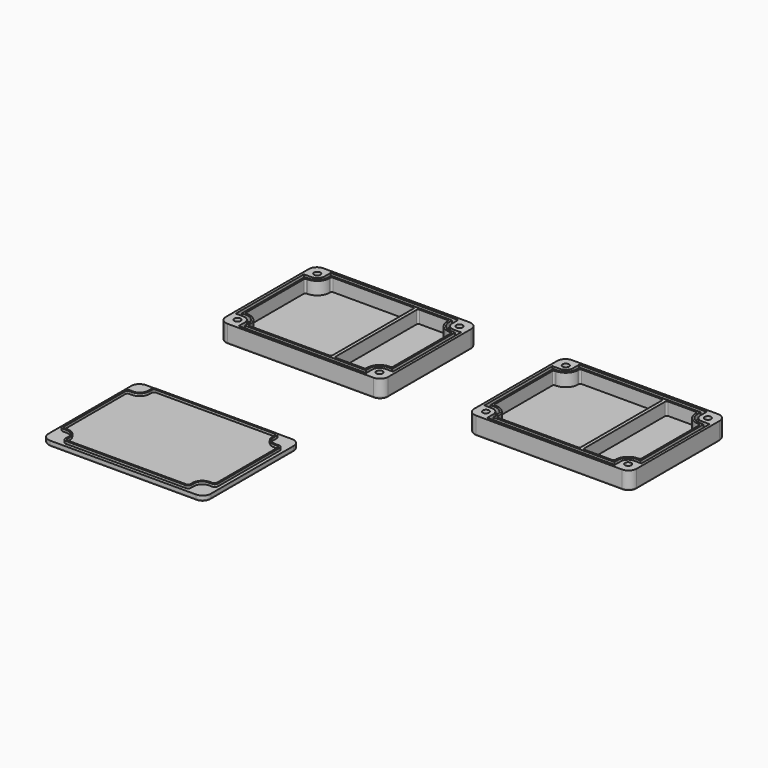
from build123d import *

# Parameters (mm, degrees)
F0_R      = 1.95
F1_DEPTH  = 11
F2_DEPTH  = 8
F3_DEPTH  = 3.2
F4_R      = 1.25
F5_DEPTH  = 3.2
F4_W      = 2
F4_H      = 66.4
F6_DEPTH  = 4.7
F4_R_2    = 2.75
F7_DEPTH  = 3.2
F8_DEPTH  = 3.2
F9_DEPTH  = 3.2
F10_R     = 1
F10_2_R   = 1
F12_R     = 3.65
F12_R_2   = 1.95
F13_DEPTH = 3.7
F17_DEPTH = 1.5
F18_DEPTH = 1.5
F19_R     = 2


# Not quite as in the source:
# - two fillets or chamfers of one size are made in one step


with BuildPart() as f1:
    # F0 (on Top) → F1 (new body)
    with BuildSketch(Plane.XY):
        with BuildLine():
            Line((56.8, 36.8), (-32.8, 36.8))
            ThreePointArc((-32.8, 36.8), (-36.3355339059, 35.3355339059), (-37.8, 31.8))
            Line((-37.8, 31.8), (-37.8, -31.8))
            ThreePointArc((-37.8, -31.8), (-36.3355339059, -35.3355339059), (-32.8, -36.8))
            Line((-32.8, -36.8), (56.8, -36.8))
            ThreePointArc((56.8, -36.8), (60.3355339059, -35.3355339059), (61.8, -31.8))
            Line((61.8, -31.8), (61.8, 31.8))
            ThreePointArc((61.8, 31.8), (60.3355339059, 35.3355339059), (56.8, 36.8))
        make_face()
        with Locations((-31.6, -30.6)):
            Circle(F0_R, mode=Mode.SUBTRACT)
        with Locations((55.6, -30.6)):
            Circle(F0_R, mode=Mode.SUBTRACT)
        with BuildLine():
            Line((51.1, -35.2), (-27.1, -35.2))
            Line((-27.1, -35.2), (-27.1, -30.6))
            ThreePointArc((-27.1, -30.6), (-28.4180194847, -27.4180194847), (-31.6, -26.1))
            Line((-31.6, -26.1), (-36.2, -26.1))
            Line((-36.2, -26.1), (-36.2, 26.1))
            Line((-36.2, 26.1), (-31.6, 26.1))
            ThreePointArc((-31.6, 26.1), (-28.4180194847, 27.4180194847), (-27.1, 30.6))
            Line((-27.1, 30.6), (-27.1, 35.2))
            Line((-27.1, 35.2), (51.1, 35.2))
            Line((51.1, 35.2), (51.1, 30.6))
            ThreePointArc((51.1, 30.6), (52.4180194847, 27.4180194847), (55.6, 26.1))
            Line((55.6, 26.1), (60.2, 26.1))
            Line((60.2, 26.1), (60.2, -26.1))
            Line((60.2, -26.1), (55.6, -26.1))
            ThreePointArc((55.6, -26.1), (52.4180194847, -27.4180194847), (51.1, -30.6))
            Line((51.1, -30.6), (51.1, -35.2))
        make_face(mode=Mode.SUBTRACT)
        with Locations((-31.6, 30.6)):
            Circle(F0_R, mode=Mode.SUBTRACT)
        with Locations((55.6, 30.6)):
            Circle(F0_R, mode=Mode.SUBTRACT)
    extrude(amount=F1_DEPTH)



with BuildPart() as f1b:
    # F0 (on Top) → F1, piece 2 (new body)
    with BuildSketch(Plane.XY):
        with BuildLine():
            Line((49.1, 33.1), (-25.1, 33.1))
            Line((-25.1, 33.1), (-25.1, 30.6))
            ThreePointArc((-25.1, 30.6), (-27.0038059223, 26.0038059223), (-31.6, 24.1))
            Line((-31.6, 24.1), (-34.1, 24.1))
            Line((-34.1, 24.1), (-34.1, -24.1))
            Line((-34.1, -24.1), (-31.6, -24.1))
            ThreePointArc((-31.6, -24.1), (-27.0038059223, -26.0038059223), (-25.1, -30.6))
            Line((-25.1, -30.6), (-25.1, -33.1))
            Line((-25.1, -33.1), (49.1, -33.1))
            Line((49.1, -33.1), (49.1, -30.6))
            ThreePointArc((49.1, -30.6), (51.0038059223, -26.0038059223), (55.6, -24.1))
            Line((55.6, -24.1), (58.1, -24.1))
            Line((58.1, -24.1), (58.1, 24.1))
            Line((58.1, 24.1), (55.6, 24.1))
            ThreePointArc((55.6, 24.1), (51.0038059223, 26.0038059223), (49.1, 30.6))
            Line((49.1, 30.6), (49.1, 33.1))
        make_face()
        with BuildLine():
            Line((-24, 30.6), (-24, 32))
            Line((-24, 32), (27, 32))
            Line((27, 32), (27, -32))
            Line((27, -32), (-24, -32))
            Line((-24, -32), (-24, -30.6))
            ThreePointArc((-24, -30.6), (-26.225988463, -25.225988463), (-31.6, -23))
            Line((-31.6, -23), (-33, -23))
            Line((-33, -23), (-33, 23))
            Line((-33, 23), (-31.6, 23))
            ThreePointArc((-31.6, 23), (-26.225988463, 25.225988463), (-24, 30.6))
        make_face(mode=Mode.SUBTRACT)
        with BuildLine():
            Line((55.6, 23), (57, 23))
            Line((57, 23), (57, -23))
            Line((57, -23), (55.6, -23))
            ThreePointArc((55.6, -23), (50.225988463, -25.225988463), (48, -30.6))
            Line((48, -30.6), (48, -32))
            Line((48, -32), (29, -32))
            Line((29, -32), (29, 32))
            Line((29, 32), (48, 32))
            Line((48, 32), (48, 30.6))
            ThreePointArc((48, 30.6), (50.225988463, 25.225988463), (55.6, 23))
        make_face(mode=Mode.SUBTRACT)
    extrude(amount=F1_DEPTH)


with BuildPart() as f1_1:
    add(f1.part)

    add(f1b.part)  # F2 merges F1b
    # F0 (on Top) → F2 (join)
    with BuildSketch(Plane.XY):
        with BuildLine():
            Line((-27.1, -30.6), (-27.1, -35.2))
            Line((-27.1, -35.2), (51.1, -35.2))
            Line((51.1, -35.2), (51.1, -30.6))
            ThreePointArc((51.1, -30.6), (52.4180194847, -27.4180194847), (55.6, -26.1))
            Line((55.6, -26.1), (60.2, -26.1))
            Line((60.2, -26.1), (60.2, 26.1))
            Line((60.2, 26.1), (55.6, 26.1))
            ThreePointArc((55.6, 26.1), (52.4180194847, 27.4180194847), (51.1, 30.6))
            Line((51.1, 30.6), (51.1, 35.2))
            Line((51.1, 35.2), (-27.1, 35.2))
            Line((-27.1, 35.2), (-27.1, 30.6))
            ThreePointArc((-27.1, 30.6), (-28.4180194847, 27.4180194847), (-31.6, 26.1))
            Line((-31.6, 26.1), (-36.2, 26.1))
            Line((-36.2, 26.1), (-36.2, -26.1))
            Line((-36.2, -26.1), (-31.6, -26.1))
            ThreePointArc((-31.6, -26.1), (-28.4180194847, -27.4180194847), (-27.1, -30.6))
        make_face()
        with BuildLine():
            Line((-25.1, 30.6), (-25.1, 33.1))
            Line((-25.1, 33.1), (49.1, 33.1))
            Line((49.1, 33.1), (49.1, 30.6))
            ThreePointArc((49.1, 30.6), (51.0038059223, 26.0038059223), (55.6, 24.1))
            Line((55.6, 24.1), (58.1, 24.1))
            Line((58.1, 24.1), (58.1, -24.1))
            Line((58.1, -24.1), (55.6, -24.1))
            ThreePointArc((55.6, -24.1), (51.0038059223, -26.0038059223), (49.1, -30.6))
            Line((49.1, -30.6), (49.1, -33.1))
            Line((49.1, -33.1), (-25.1, -33.1))
            Line((-25.1, -33.1), (-25.1, -30.6))
            ThreePointArc((-25.1, -30.6), (-27.0038059223, -26.0038059223), (-31.6, -24.1))
            Line((-31.6, -24.1), (-34.1, -24.1))
            Line((-34.1, -24.1), (-34.1, 24.1))
            Line((-34.1, 24.1), (-31.6, 24.1))
            ThreePointArc((-31.6, 24.1), (-27.0038059223, 26.0038059223), (-25.1, 30.6))
        make_face(mode=Mode.SUBTRACT)
    extrude(amount=F2_DEPTH)

    # F0 (on Top) → F3 (join)
    with BuildSketch(Plane.XY):
        with BuildLine():
            Line((57, -23), (57, 23))
            Line((57, 23), (55.6, 23))
            ThreePointArc((55.6, 23), (50.225988463, 25.225988463), (48, 30.6))
            Line((48, 30.6), (48, 32))
            Line((48, 32), (29, 32))
            Line((29, 32), (29, -32))
            Line((29, -32), (48, -32))
            Line((48, -32), (48, -30.6))
            ThreePointArc((48, -30.6), (50.225988463, -25.225988463), (55.6, -23))
            Line((55.6, -23), (57, -23))
        make_face()
        with BuildLine():
            Line((27, 32), (-24, 32))
            Line((-24, 32), (-24, 30.6))
            ThreePointArc((-24, 30.6), (-26.225988463, 25.225988463), (-31.6, 23))
            Line((-31.6, 23), (-33, 23))
            Line((-33, 23), (-33, -23))
            Line((-33, -23), (-31.6, -23))
            ThreePointArc((-31.6, -23), (-26.225988463, -25.225988463), (-24, -30.6))
            Line((-24, -30.6), (-24, -32))
            Line((-24, -32), (27, -32))
            Line((27, -32), (27, 32))
        make_face()
    extrude(amount=F3_DEPTH)

    # F10#2
    f10_2_edges = [f1_1.edges().sort_by_distance(p)[0] for p in [
        (-24, 32, 7.1),
        (27, 32, 7.1),
        (27, -32, 7.1),
        (-24, -32, 7.1),
        (-33, -23, 7.1),
        (-33, 23, 7.1),
        (57, 23, 7.1),
        (57, -23, 7.1),
        (48, -32, 7.1),
        (29, -32, 7.1),
        (29, 32, 7.1),
        (48, 32, 7.1),
        (12, 36.8, 0),
        (-36.335534, 35.335534, 0),
        (-37.8, 0, 0),
        (-36.335534, -35.335534, 0),
        (12, -36.8, 0),
        (60.335534, -35.335534, 0),
        (61.8, 0, 0),
        (60.335534, 35.335534, 0),
    ]]
    fillet(f10_2_edges, radius=F10_2_R)

    # F12 (on face) → F13 (cut)
    with BuildSketch(Plane(origin=(0, 0, 0), x_dir=(1, 0, 0), z_dir=(0, 0, -1))):
        with Locations((55.6, -30.6)):
            Circle(F12_R)
        with Locations((55.6, -30.6)):
            Circle(F12_R_2, mode=Mode.SUBTRACT)
        with Locations((55.6, 30.6)):
            Circle(F12_R)
        with Locations((55.6, 30.6)):
            Circle(F12_R_2, mode=Mode.SUBTRACT)
        with Locations((-31.6, -30.6)):
            Circle(F12_R)
        with Locations((-31.6, -30.6)):
            Circle(F12_R_2, mode=Mode.SUBTRACT)
        with Locations((-31.6, 30.6)):
            Circle(F12_R)
        with Locations((-31.6, 30.6)):
            Circle(F12_R_2, mode=Mode.SUBTRACT)
    extrude(amount=-F13_DEPTH, mode=Mode.SUBTRACT)


with BuildPart() as f5:
    # F4 (on Top) → F5 (new body)
    with BuildSketch(Plane.XY):
        with BuildLine():
            Line((56.8, -99.2), (-32.8, -99.2))
            ThreePointArc((-32.8, -99.2), (-36.3355339059, -100.6644660941), (-37.8, -104.2))
            Line((-37.8, -104.2), (-37.8, -167.8))
            ThreePointArc((-37.8, -167.8), (-36.3355339059, -171.3355339059), (-32.8, -172.8))
            Line((-32.8, -172.8), (56.8, -172.8))
            ThreePointArc((56.8, -172.8), (60.3355339059, -171.3355339059), (61.8, -167.8))
            Line((61.8, -167.8), (61.8, -104.2))
            ThreePointArc((61.8, -104.2), (60.3355339059, -100.6644660941), (56.8, -99.2))
        make_face()
        with Locations((-31.6, -166.6)):
            Circle(F4_R, mode=Mode.SUBTRACT)
        with Locations((55.6, -166.6)):
            Circle(F4_R, mode=Mode.SUBTRACT)
        with BuildLine():
            Line((-27, -105.4), (-27, -100.9))
            Line((-27, -100.9), (51, -100.9))
            Line((51, -100.9), (51.0491758988, -100.9))
            ThreePointArc((51.0491758988, -100.9), (51.0245188805, -100.9250729028), (51, -100.9502809077))
            Line((51, -100.9502809077), (51, -105.4))
            ThreePointArc((51, -105.4), (52.3473088065, -108.6526911935), (55.6, -110))
            Line((55.6, -110), (60.0497190923, -110))
            ThreePointArc((60.0497190923, -110), (60.0749270972, -109.9754811195), (60.1, -109.9508241012))
            Line((60.1, -109.9508241012), (60.1, -110))
            Line((60.1, -110), (60.1, -162))
            Line((60.1, -162), (60.1, -162.0491758988))
            ThreePointArc((60.1, -162.0491758988), (60.0749270972, -162.0245188805), (60.0497190923, -162))
            Line((60.0497190923, -162), (55.6, -162))
            ThreePointArc((55.6, -162), (52.3473088065, -163.3473088065), (51, -166.6))
            Line((51, -166.6), (51, -171.0497190923))
            ThreePointArc((51, -171.0497190923), (51.0245188805, -171.0749270972), (51.0491758988, -171.1))
            Line((51.0491758988, -171.1), (51, -171.1))
            Line((51, -171.1), (-27, -171.1))
            Line((-27, -171.1), (-27.0491758988, -171.1))
            ThreePointArc((-27.0491758988, -171.1), (-27.0245188805, -171.0749270972), (-27, -171.0497190923))
            Line((-27, -171.0497190923), (-27, -166.6))
            ThreePointArc((-27, -166.6), (-28.3473088065, -163.3473088065), (-31.6, -162))
            Line((-31.6, -162), (-36.0497190923, -162))
            ThreePointArc((-36.0497190923, -162), (-36.0749270972, -162.0245188805), (-36.1, -162.0491758988))
            Line((-36.1, -162.0491758988), (-36.1, -162))
            Line((-36.1, -162), (-36.1, -110))
            Line((-36.1, -110), (-31.6, -110))
            ThreePointArc((-31.6, -110), (-28.3473088065, -108.6526911935), (-27, -105.4))
        make_face(mode=Mode.SUBTRACT)
        with Locations((-31.6, -105.4)):
            Circle(F4_R, mode=Mode.SUBTRACT)
        with Locations((55.6, -105.4)):
            Circle(F4_R, mode=Mode.SUBTRACT)
    extrude(amount=F5_DEPTH)



with BuildPart() as f5b:
    # F4 (on Top) → F5, piece 2 (new body)
    with BuildSketch(Plane.XY):
        with Locations((28, -136)):
            Rectangle(F4_W, F4_H)
    extrude(amount=F5_DEPTH)


with BuildPart() as f5_1:
    add(f5.part)

    add(f5b.part)  # F6 merges F5b
    # F4 (on Top) → F6 (join)
    with BuildSketch(Plane.XY):
        with BuildLine():
            Line((51, -100.9), (-27, -100.9))
            Line((-27, -100.9), (-27, -105.4))
            ThreePointArc((-27, -105.4), (-28.3473088065, -108.6526911935), (-31.6, -110))
            Line((-31.6, -110), (-36.1, -110))
            Line((-36.1, -110), (-36.1, -162))
            Line((-36.1, -162), (-36.0497190923, -162))
            Line((-36.0497190923, -162), (-31.6, -162))
            ThreePointArc((-31.6, -162), (-28.3473088065, -163.3473088065), (-27, -166.6))
            Line((-27, -166.6), (-27, -171.0497190923))
            Line((-27, -171.0497190923), (-27, -171.1))
            Line((-27, -171.1), (51, -171.1))
            Line((51, -171.1), (51, -171.0497190923))
            Line((51, -171.0497190923), (51, -166.6))
            ThreePointArc((51, -166.6), (52.3473088065, -163.3473088065), (55.6, -162))
            Line((55.6, -162), (60.0497190923, -162))
            Line((60.0497190923, -162), (60.1, -162))
            Line((60.1, -162), (60.1, -110))
            Line((60.1, -110), (60.0497190923, -110))
            Line((60.0497190923, -110), (55.6, -110))
            ThreePointArc((55.6, -110), (52.3473088065, -108.6526911935), (51, -105.4))
            Line((51, -105.4), (51, -100.9502809077))
            Line((51, -100.9502809077), (51, -100.9))
        make_face()
        with BuildLine():
            Line((-25.2, -105.4), (-25.2, -102.8))
            Line((-25.2, -102.8), (27, -102.8))
            Line((27, -102.8), (29, -102.8))
            Line((29, -102.8), (49.2, -102.8))
            Line((49.2, -102.8), (49.2, -105.4))
            ThreePointArc((49.2, -105.4), (51.0745166004, -109.9254833996), (55.6, -111.8))
            Line((55.6, -111.8), (58.2, -111.8))
            Line((58.2, -111.8), (58.2, -160.2))
            Line((58.2, -160.2), (55.6, -160.2))
            ThreePointArc((55.6, -160.2), (51.0745166004, -162.0745166004), (49.2, -166.6))
            Line((49.2, -166.6), (49.2, -169.2))
            Line((49.2, -169.2), (29, -169.2))
            Line((29, -169.2), (27, -169.2))
            Line((27, -169.2), (-25.2, -169.2))
            Line((-25.2, -169.2), (-25.2, -166.6))
            ThreePointArc((-25.2, -166.6), (-27.0745166004, -162.0745166004), (-31.6, -160.2))
            Line((-31.6, -160.2), (-34.2, -160.2))
            Line((-34.2, -160.2), (-34.2, -111.8))
            Line((-34.2, -111.8), (-31.6, -111.8))
            ThreePointArc((-31.6, -111.8), (-27.0745166004, -109.9254833996), (-25.2, -105.4))
        make_face(mode=Mode.SUBTRACT)
    extrude(amount=F6_DEPTH)

    # F4 (on Top) → F7 (join)
    with BuildSketch(Plane.XY):
        with Locations((-31.6, -105.4)):
            Circle(F4_R)
        with Locations((55.6, -105.4)):
            Circle(F4_R)
        with Locations((-31.6, -166.6)):
            Circle(F4_R)
        with Locations((55.6, -166.6)):
            Circle(F4_R)
        with BuildLine():
            Line((49.2, -102.8), (29, -102.8))
            Line((29, -102.8), (29, -169.2))
            Line((29, -169.2), (49.2, -169.2))
            Line((49.2, -169.2), (49.2, -166.6))
            ThreePointArc((49.2, -166.6), (51.0745166004, -162.0745166004), (55.6, -160.2))
            Line((55.6, -160.2), (58.2, -160.2))
            Line((58.2, -160.2), (58.2, -111.8))
            Line((58.2, -111.8), (55.6, -111.8))
            ThreePointArc((55.6, -111.8), (51.0745166004, -109.9254833996), (49.2, -105.4))
            Line((49.2, -105.4), (49.2, -102.8))
        make_face()
        with BuildLine():
            Line((27, -102.8), (-25.2, -102.8))
            Line((-25.2, -102.8), (-25.2, -105.4))
            ThreePointArc((-25.2, -105.4), (-27.0745166004, -109.9254833996), (-31.6, -111.8))
            Line((-31.6, -111.8), (-34.2, -111.8))
            Line((-34.2, -111.8), (-34.2, -160.2))
            Line((-34.2, -160.2), (-31.6, -160.2))
            ThreePointArc((-31.6, -160.2), (-27.0745166004, -162.0745166004), (-25.2, -166.6))
            Line((-25.2, -166.6), (-25.2, -169.2))
            Line((-25.2, -169.2), (27, -169.2))
            Line((27, -169.2), (27, -102.8))
        make_face()
        with Locations((-20, -156)):
            Circle(F4_R_2, mode=Mode.SUBTRACT)
        with Locations((20, -156)):
            Circle(F4_R_2, mode=Mode.SUBTRACT)
        with Locations((-20, -116)):
            Circle(F4_R_2, mode=Mode.SUBTRACT)
        with Locations((20, -116)):
            Circle(F4_R_2, mode=Mode.SUBTRACT)
    extrude(amount=F7_DEPTH)

    # F4 (on Top) → F8 (join, through all)
    with BuildSketch(Plane.XY):
        with Locations((-20, -116)):
            Circle(F4_R_2)
        with Locations((-20, -116)):
            Circle(F4_R, mode=Mode.SUBTRACT)
        with Locations((-20, -156)):
            Circle(F4_R_2)
        with Locations((-20, -156)):
            Circle(F4_R, mode=Mode.SUBTRACT)
        with Locations((20, -156)):
            Circle(F4_R_2)
        with Locations((20, -156)):
            Circle(F4_R, mode=Mode.SUBTRACT)
        with Locations((20, -116)):
            Circle(F4_R_2)
        with Locations((20, -116)):
            Circle(F4_R, mode=Mode.SUBTRACT)
    extrude(amount=F8_DEPTH)

    # F4 (on Top) → F9 (join, through all)
    with BuildSketch(Plane.XY):
        with Locations((-20, -116)):
            Circle(F4_R)
        with Locations((20, -116)):
            Circle(F4_R)
        with Locations((20, -156)):
            Circle(F4_R)
        with Locations((-20, -156)):
            Circle(F4_R)
    extrude(amount=F9_DEPTH)

    # F10
    f10_edges = [f5_1.edges().sort_by_distance(p)[0] for p in [
        (49.2, -102.8, 3.95),
        (58.2, -111.8, 3.95),
        (58.2, -160.2, 3.95),
        (49.2, -169.2, 3.95),
        (-25.2, -102.8, 3.95),
        (-34.2, -111.8, 3.95),
        (-25.2, -169.2, 3.95),
        (-34.2, -160.2, 3.95),
        (61.8, -136, 0),
        (60.335534, -171.335534, 0),
        (60.335534, -100.664466, 0),
        (12, -99.2, 0),
        (-36.335534, -100.664466, 0),
        (-37.8, -136, 0),
        (-36.335534, -171.335534, 0),
        (12, -172.8, 0),
    ]]
    fillet(f10_edges, radius=F10_R)

    # F16 (on face) → F17 (cut, through all)
    with BuildSketch(Plane.XY.offset(4.7)):
        with BuildLine():
            Line((-36.1, -110), (-36.1, -162))
            Line((-36.1, -162), (-31.6, -162))
            ThreePointArc((-31.6, -162), (-28.3473088065, -163.3473088065), (-27, -166.6))
            Line((-27, -166.6), (-27, -171.1))
            Line((-27, -171.1), (51, -171.1))
            Line((51, -171.1), (51, -166.6))
            ThreePointArc((51, -166.6), (52.3473088065, -163.3473088065), (55.6, -162))
            Line((55.6, -162), (60.1, -162))
            Line((60.1, -162), (60.1, -110))
            Line((60.1, -110), (55.6, -110))
            ThreePointArc((55.6, -110), (52.3473088065, -108.6526911935), (51, -105.4))
            Line((51, -105.4), (51, -100.9))
            Line((51, -100.9), (-27, -100.9))
            Line((-27, -100.9), (-27, -105.4))
            ThreePointArc((-27, -105.4), (-28.3473088065, -108.6526911935), (-31.6, -110))
            Line((-31.6, -110), (-36.1, -110))
        make_face()
        with BuildLine():
            ThreePointArc((-31.6, -110.4), (-28.0644660941, -108.9355339059), (-26.6, -105.4))
            Line((-26.6, -105.4), (-26.6, -101.3))
            Line((-26.6, -101.3), (50.6, -101.3))
            Line((50.6, -101.3), (50.6, -105.4))
            ThreePointArc((50.6, -105.4), (52.0644660941, -108.9355339059), (55.6, -110.4))
            Line((55.6, -110.4), (59.7, -110.4))
            Line((59.7, -110.4), (59.7, -161.6))
            Line((59.7, -161.6), (55.6, -161.6))
            ThreePointArc((55.6, -161.6), (52.0644660941, -163.0644660941), (50.6, -166.6))
            Line((50.6, -166.6), (50.6, -170.7))
            Line((50.6, -170.7), (-26.6, -170.7))
            Line((-26.6, -170.7), (-26.6, -166.6))
            ThreePointArc((-26.6, -166.6), (-28.0644660941, -163.0644660941), (-31.6, -161.6))
            Line((-31.6, -161.6), (-35.7, -161.6))
            Line((-35.7, -161.6), (-35.7, -110.4))
            Line((-35.7, -110.4), (-31.6, -110.4))
        make_face(mode=Mode.SUBTRACT)
    extrude(amount=-F17_DEPTH, mode=Mode.SUBTRACT)

    # F16 (on face) → F18 (cut, through all)
    with BuildSketch(Plane.XY.offset(4.7)):
        with BuildLine():
            ThreePointArc((58.7, -112.8), (58.2606601718, -111.7393398282), (57.2, -111.3))
            Line((57.2, -111.3), (55.6, -111.3))
            ThreePointArc((55.6, -111.3), (51.428069991, -109.571930009), (49.7, -105.4))
            Line((49.7, -105.4), (49.7, -103.8))
            ThreePointArc((49.7, -103.8), (49.2606601718, -102.7393398282), (48.2, -102.3))
            Line((48.2, -102.3), (-24.2, -102.3))
            ThreePointArc((-24.2, -102.3), (-25.2606601718, -102.7393398282), (-25.7, -103.8))
            Line((-25.7, -103.8), (-25.7, -105.4))
            ThreePointArc((-25.7, -105.4), (-27.428069991, -109.571930009), (-31.6, -111.3))
            Line((-31.6, -111.3), (-33.2, -111.3))
            ThreePointArc((-33.2, -111.3), (-34.2606601718, -111.7393398282), (-34.7, -112.8))
            Line((-34.7, -112.8), (-34.7, -159.2))
            ThreePointArc((-34.7, -159.2), (-34.2606601718, -160.2606601718), (-33.2, -160.7))
            Line((-33.2, -160.7), (-31.6, -160.7))
            ThreePointArc((-31.6, -160.7), (-27.428069991, -162.428069991), (-25.7, -166.6))
            Line((-25.7, -166.6), (-25.7, -168.2))
            ThreePointArc((-25.7, -168.2), (-25.2606601718, -169.2606601718), (-24.2, -169.7))
            Line((-24.2, -169.7), (48.2, -169.7))
            ThreePointArc((48.2, -169.7), (49.2606601718, -169.2606601718), (49.7, -168.2))
            Line((49.7, -168.2), (49.7, -166.6))
            ThreePointArc((49.7, -166.6), (51.428069991, -162.428069991), (55.6, -160.7))
            Line((55.6, -160.7), (57.2, -160.7))
            ThreePointArc((57.2, -160.7), (58.2606601718, -160.2606601718), (58.7, -159.2))
            Line((58.7, -159.2), (58.7, -112.8))
        make_face()
        with BuildLine():
            ThreePointArc((-25.2, -103.8), (-24.9071067812, -103.0928932188), (-24.2, -102.8))
            Line((-24.2, -102.8), (48.2, -102.8))
            ThreePointArc((48.2, -102.8), (48.9071067812, -103.0928932188), (49.2, -103.8))
            Line((49.2, -103.8), (49.2, -105.4))
            ThreePointArc((49.2, -105.4), (51.0745166004, -109.9254833996), (55.6, -111.8))
            Line((55.6, -111.8), (57.2, -111.8))
            ThreePointArc((57.2, -111.8), (57.9071067812, -112.0928932188), (58.2, -112.8))
            Line((58.2, -112.8), (58.2, -159.2))
            ThreePointArc((58.2, -159.2), (57.9071067812, -159.9071067812), (57.2, -160.2))
            Line((57.2, -160.2), (55.6, -160.2))
            ThreePointArc((55.6, -160.2), (51.0745166004, -162.0745166004), (49.2, -166.6))
            Line((49.2, -166.6), (49.2, -168.2))
            ThreePointArc((49.2, -168.2), (48.9071067812, -168.9071067812), (48.2, -169.2))
            Line((48.2, -169.2), (-24.2, -169.2))
            ThreePointArc((-24.2, -169.2), (-24.9071067812, -168.9071067812), (-25.2, -168.2))
            Line((-25.2, -168.2), (-25.2, -166.6))
            ThreePointArc((-25.2, -166.6), (-27.0745166004, -162.0745166004), (-31.6, -160.2))
            Line((-31.6, -160.2), (-33.2, -160.2))
            ThreePointArc((-33.2, -160.2), (-33.9071067812, -159.9071067812), (-34.2, -159.2))
            Line((-34.2, -159.2), (-34.2, -112.8))
            ThreePointArc((-34.2, -112.8), (-33.9071067812, -112.0928932188), (-33.2, -111.8))
            Line((-33.2, -111.8), (-31.6, -111.8))
            ThreePointArc((-31.6, -111.8), (-27.0745166004, -109.9254833996), (-25.2, -105.4))
            Line((-25.2, -105.4), (-25.2, -103.8))
        make_face(mode=Mode.SUBTRACT)
    extrude(amount=-F18_DEPTH, mode=Mode.SUBTRACT)

    # F19
    f19_edges = [f5_1.edges().sort_by_distance(p)[0] for p in [
        (59.7, -161.6, 3.95),
        (50.6, -170.7, 3.95),
        (-26.6, -170.7, 3.95),
        (-35.7, -161.6, 3.95),
        (-35.7, -110.4, 3.95),
        (-26.6, -101.3, 3.95),
        (50.6, -101.3, 3.95),
        (59.7, -110.4, 3.95),
    ]]
    fillet(f19_edges, radius=F19_R)


with BuildPart() as f23_1:
    # F23: copy of F1
    add(f1_1.part.moved(Location((152.4, 0, 0))))


solid = Compound([f1_1.part, f5_1.part, f23_1.part])
